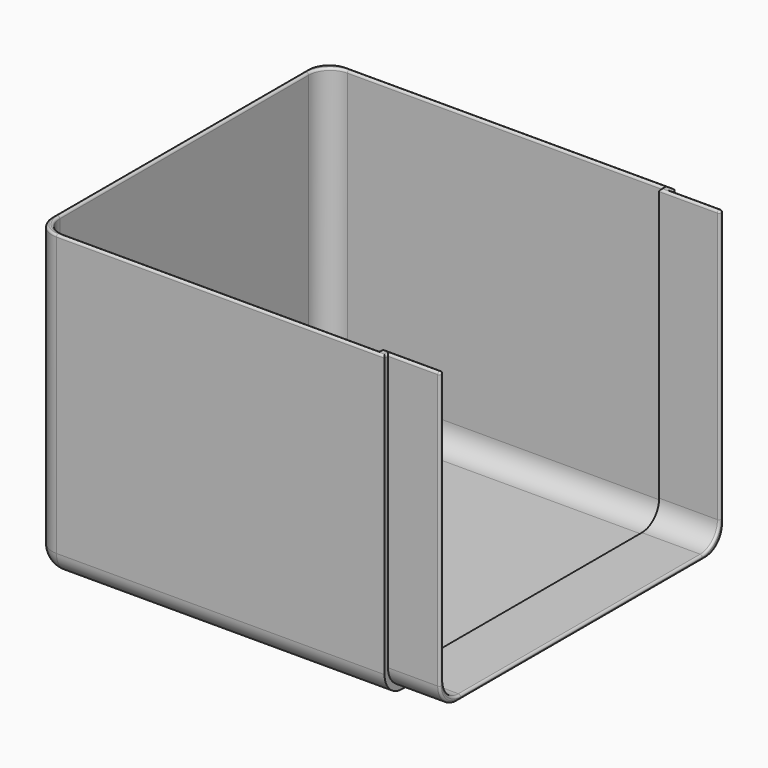
from build123d import *

# Parameters (mm, degrees)
F0_W     = 81
F0_H     = 84
F1_DEPTH = 70
F3_DEPTH = 69
F5_DEPTH = 2
F7_DEPTH = 14
F8_R     = 5
F9_R     = 0.49999


# Not quite as in the source:
# - a fillet or chamfer is up to 0.001 mm smaller than in the source, because OpenCascade refuses the exact size


with BuildPart() as f1:
    # F0 (on Top) → F1 (new body)
    with BuildSketch(Plane.XY):
        Rectangle(F0_W, F0_H)
    extrude(amount=F1_DEPTH)

    # F2 (on face) → F3 (cut)
    with BuildSketch(Plane.XY.offset(70)):
        Polygon((38.5, 41), (-39.5, 41), (-39.5, 20.586034283), (-39.5, -41), (38.5, -41), (38.5, -37.5405208561), align=None)
    extrude(amount=-F3_DEPTH, mode=Mode.SUBTRACT)

    # F4 (on face) → F5 (cut)
    with BuildSketch(Plane.YZ.offset(40.5)):
        Polygon((40, 2), (40, 70), (-40, 70), (-40, 42.2970801592), (-40, 2), align=None)
    extrude(amount=-F5_DEPTH, mode=Mode.SUBTRACT)

    # F6 (on face) → F7 (join)
    with BuildSketch(Plane(origin=(38.5, 0, 0), x_dir=(0, -1, 0), z_dir=(-1, 0, 0))):
        Polygon((41, 1), (41, 70), (40, 70), (40, 2), (-40, 2), (-40, 70), (-41, 70), (-41, 1), align=None)
    extrude(amount=-F7_DEPTH)

    # F8
    f8_edges = [f1.edges().sort_by_distance(p)[0] for p in [
        (-0.5, 41, 1),
        (-39.5, 0, 1),
        (-0.5, -41, 1),
        (0, 42, 0),
        (-40.5, 0, 0),
        (0, -42, 0),
        (-40.5, -42, 35),
        (-40.5, 42, 35),
        (-39.5, 41, 35.5),
        (-39.5, -41, 35.5),
        (46.5, 41, 1),
        (46.5, -41, 1),
        (45.5, -40, 2),
        (45.5, 40, 2),
    ]]
    fillet(f8_edges, radius=F8_R)

    # F9 (radius 0.5 in the source; OpenCascade refuses exactly that, so slightly less here)
    f9_edges = [f1.edges().sort_by_distance(p)[0] for p in [
        (2.5, 42, 70),
        (-39.035534, 40.535534, 70),
        (40.5, 41.5, 70),
        (-40.5, 0, 70),
        (46.5, 41, 70),
        (-39.035534, -40.535534, 70),
        (52.5, 40.5, 70),
        (2.5, -42, 70),
        (45.5, 40, 70),
        (40.5, -41.5, 70),
        (38.5, 40.5, 70),
        (46.5, -41, 70),
        (2, 41, 70),
        (52.5, -40.5, 70),
        (-38.035534, 39.535534, 70),
        (45.5, -40, 70),
        (-39.5, 0, 70),
        (38.5, -40.5, 70),
        (-38.035534, -39.535534, 70),
        (2, -41, 70),
        (52.5, -41, 38),
        (52.5, -39.535534, 2.464466),
        (52.5, 0, 1),
        (52.5, -40, 38.5),
        (52.5, 39.535534, 2.464466),
        (52.5, -38.535534, 3.464466),
        (52.5, 41, 38),
        (52.5, 0, 2),
        (52.5, 38.535534, 3.464466),
        (52.5, 40, 38.5),
    ]]
    fillet(f9_edges, radius=F9_R)


solid = f1.part
